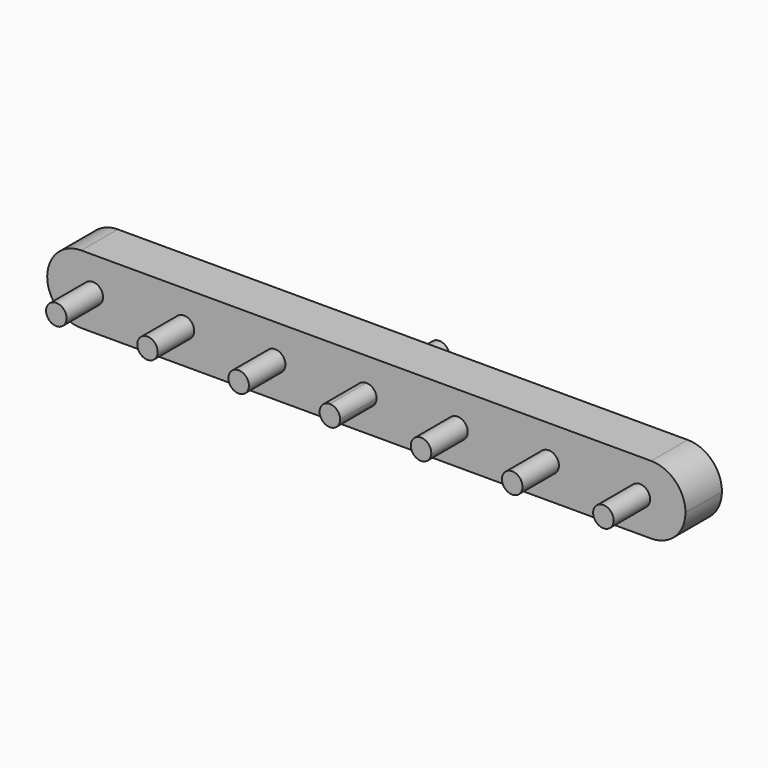
from build123d import *

# Parameters (mm, degrees)
F0_R     = 2.8575
F1_DEPTH = 12.7
F2_DEPTH = 25.4
F3_R     = 2.8575
F4_DEPTH = 12.7
F5_R     = 9.52499


# Not quite as in the source:
# - a fillet or chamfer is up to 0.001 mm smaller than in the source, because OpenCascade refuses the exact size
# - a feature names something its author has since deleted; it is built from what else it names


with BuildPart() as f1:
    # F0 (on Front) → F1 (new body)
    with BuildSketch(Plane.XZ):
        Polygon((-88.9, -9.525), (88.9, -9.525), (88.9, 9.525), (0, 9.525), (-88.9, 9.525), align=None)
        with Locations((-76.2, 0)):
            Circle(F0_R, mode=Mode.SUBTRACT)
        with Locations((-50.8, 0)):
            Circle(F0_R, mode=Mode.SUBTRACT)
        with Locations((-25.4, 0)):
            Circle(F0_R, mode=Mode.SUBTRACT)
        with BuildLine():
            ThreePointArc((2.8575, 0), (-2.0205576272, -2.0205576272), (0, 2.8575))
            ThreePointArc((0, 2.8575), (2.0205576272, 2.0205576272), (2.8575, 0))
        make_face(mode=Mode.SUBTRACT)
        with Locations((25.4, 0)):
            Circle(F0_R, mode=Mode.SUBTRACT)
        with Locations((50.8, 0)):
            Circle(F0_R, mode=Mode.SUBTRACT)
        with Locations((76.2, 0)):
            Circle(F0_R, mode=Mode.SUBTRACT)
    extrude(amount=F1_DEPTH)

    # F0 (on Front) → F2 (join)
    with BuildSketch(Plane.XZ):
        with BuildLine():
            ThreePointArc((2.8575, 0), (2.0205576272, 2.0205576272), (0, 2.8575))
            ThreePointArc((0, 2.8575), (-2.0205576272, -2.0205576272), (2.8575, 0))
        make_face()
        with Locations((-76.2, 0)):
            Circle(F0_R)
        with Locations((-50.8, 0)):
            Circle(F0_R)
        with Locations((-25.4, 0)):
            Circle(F0_R)
        with Locations((25.4, 0)):
            Circle(F0_R)
        with Locations((50.8, 0)):
            Circle(F0_R)
        with Locations((76.2, 0)):
            Circle(F0_R)
    extrude(amount=F2_DEPTH)

    # F3 (on face) → F4 (join)
    with BuildSketch(Plane(origin=(0, 0, 0), x_dir=(-1, 0, 0), z_dir=(0, 1, 0))):
        Circle(F3_R)
    extrude(amount=F4_DEPTH)

    # F5 (radius 9.525 in the source; OpenCascade refuses exactly that, so slightly less here)
    f5_edges = [f1.edges().sort_by_distance(p)[0] for p in [
        (88.9, -6.35, 9.525),
        (88.9, -6.35, -9.525),
        (-88.9, -6.35, -9.525),
        (-88.9, -6.35, 9.525),
    ]]
    fillet(f5_edges, radius=F5_R)


solid = f1.part
